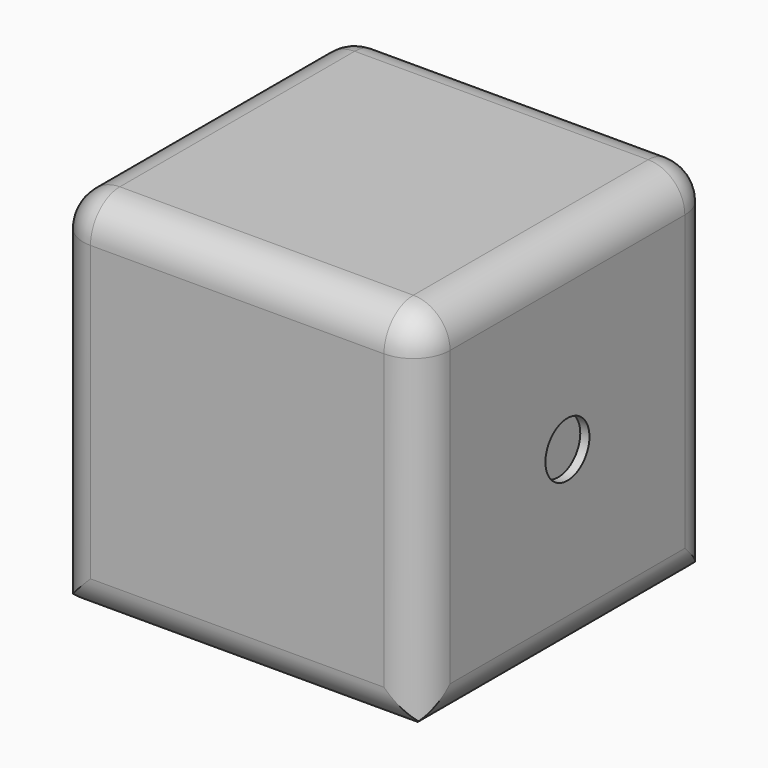
from build123d import *

# Parameters (mm, degrees)
F0_W         = 50.8
F0_H         = 50.8
F1_DEPTH     = 50.8
F2_R         = 5.08
F3_R         = 5.08
F4_T1_DEPTH  = 58.42
F4_T3_DEPTH  = 76.2
F4_T5_DEPTH  = 40.64
F4_S9_W      = 5.08
F4_S9_H      = 5.08
F4_T10_DEPTH = 5.08
F4_S15_W     = 5.08
F4_S15_H     = 5.08
F4_T16_DEPTH = 5.08
F4_T20_ANGLE = 90
F4_T22_ANGLE = 90
F5_T1_DEPTH  = 66.04
F6_T1_DEPTH  = 66.04
F7_R         = 3.81
F8_DEPTH     = 1.27


# Not quite as in the source:
# - a fillet or chamfer that OpenCascade refuses, or shapes differently, is made with other operations: its cross-section is extruded or revolved along the edge and cut away or added


with BuildPart() as f1:
    # F0 (on Front) → F1 (new body)
    with BuildSketch(Plane.XZ):
        with Locations((25.4, 25.4)):
            Rectangle(F0_W, F0_H)
    extrude(amount=F1_DEPTH)

    # F2
    f2_edges = [f1.edges().sort_by_distance(p)[0] for p in [
        (25.4, -50.8, 50.8),
    ]]
    fillet(f2_edges, radius=F2_R)

    # F3
    f3_edges = [f1.edges().sort_by_distance(p)[0] for p in [
        (25.4, 0, 50.8),
        (0, 0, 25.4),
        (25.4, 0, 0),
        (50.8, 0, 25.4),
    ]]
    fillet(f3_edges, radius=F3_R)

    # F4: fillet of radius 5.08 on 4 edges, made by hand

    # F4_s2 → F4_t1 (cut)
    with BuildSketch(Plane.XY.offset(-12.7)):
        with BuildLine():
            ThreePointArc((0, -45.72), (1.4878975516, -49.3121024484), (5.08, -50.8))
            Line((5.08, -50.8), (0, -50.8))
            Line((0, -50.8), (0, -45.72))
        make_face()
        with BuildLine():
            ThreePointArc((45.72, -50.8), (49.3121024484, -49.3121024484), (50.8, -45.72))
            Line((50.8, -45.72), (50.8, -50.8))
            Line((50.8, -50.8), (45.72, -50.8))
        make_face()
    extrude(amount=F4_T1_DEPTH, mode=Mode.SUBTRACT)

    # F4_s4 → F4_t3 (cut)
    with BuildSketch(Plane.YZ.offset(-12.7)):
        with BuildLine():
            ThreePointArc((-45.72, 0), (-49.3121024484, 1.4878975516), (-50.8, 5.08))
            Line((-50.8, 5.08), (-50.8, 0))
            Line((-50.8, 0), (-45.72, 0))
        make_face()
    extrude(amount=F4_T3_DEPTH, mode=Mode.SUBTRACT)

    # F4_s6 → F4_t5 (cut)
    with BuildSketch(Plane.XZ.offset(5.08)):
        with BuildLine():
            ThreePointArc((45.72, 50.8), (49.3121024484, 49.3121024484), (50.8, 45.72))
            Line((50.8, 45.72), (50.8, 50.8))
            Line((50.8, 50.8), (45.72, 50.8))
        make_face()
        with BuildLine():
            ThreePointArc((0, 45.72), (1.4878975516, 49.3121024484), (5.08, 50.8))
            Line((5.08, 50.8), (0, 50.8))
            Line((0, 50.8), (0, 45.72))
        make_face()
    extrude(amount=F4_T5_DEPTH, mode=Mode.SUBTRACT)


with BuildPart() as f4_tool8:
    # F4_s9 → F4_t10 (new body)
    with BuildSketch(Plane.XY.offset(45.72)):
        with Locations((48.26, -2.54)):
            Rectangle(F4_S9_W, F4_S9_H)
    extrude(amount=F4_T10_DEPTH)

    # F4_s11 → F4_t12 (revolve, cut)
    with BuildSketch(Plane(origin=(45.72, -5.08, 45.72), x_dir=(-0.7071067812, -0.7071067812, 0), z_dir=(-0.7071067812, 0.7071067812, 0))):
        with BuildLine():
            ThreePointArc((0, -5.08), (5.08, 0), (0, 5.08))
            Line((0, 5.08), (0, -5.08))
        make_face()
    revolve(axis=Axis((45.72, -5.08, 45.72), (0, 0, 1)), mode=Mode.SUBTRACT)


with BuildPart() as f1_1:
    add(f1.part)

    # F4_t7: cut F4_tool8
    add(f4_tool8.part, mode=Mode.SUBTRACT)


with BuildPart() as f4_tool14:
    # F4_s15 → F4_t16 (new body)
    with BuildSketch(Plane.YZ.offset(5.08)):
        with Locations((-2.54, 48.26)):
            Rectangle(F4_S15_W, F4_S15_H)
    extrude(amount=-F4_T16_DEPTH)

    # F4_s17 → F4_t18 (revolve, cut)
    with BuildSketch(Plane(origin=(5.08, -5.08, 45.72), x_dir=(0, -0.7071067812, -0.7071067812), z_dir=(0, 0.7071067812, -0.7071067812))):
        with BuildLine():
            ThreePointArc((0, -5.08), (5.08, 0), (0, 5.08))
            Line((0, 5.08), (0, -5.08))
        make_face()
    revolve(axis=Axis((5.08, -5.08, 45.72), (-1, 0, 0)), mode=Mode.SUBTRACT)


with BuildPart() as f1_2:
    add(f1_1.part)

    # F4_t13: cut F4_tool14
    add(f4_tool14.part, mode=Mode.SUBTRACT)

    # F4_s19 → F4_t20 (revolve, cut)
    with BuildSketch(Plane.XZ.offset(45.72)):
        with BuildLine():
            ThreePointArc((45.72, 50.8), (49.3121024484, 49.3121024484), (50.8, 45.72))
            Line((50.8, 45.72), (50.8, 50.8))
            Line((50.8, 50.8), (45.72, 50.8))
        make_face()
    revolve(axis=Axis((50.8, -45.72, 45.72), (1, 0, 0)), revolution_arc=F4_T20_ANGLE, mode=Mode.SUBTRACT)

    # F4_s21 → F4_t22 (revolve, cut)
    with BuildSketch(Plane.XZ.offset(45.72)):
        with BuildLine():
            ThreePointArc((0, 45.72), (1.4878975516, 49.3121024484), (5.08, 50.8))
            Line((5.08, 50.8), (0, 50.8))
            Line((0, 50.8), (0, 45.72))
        make_face()
    revolve(axis=Axis((0, -45.72, 45.72), (1, 0, 0)), revolution_arc=F4_T22_ANGLE, mode=Mode.SUBTRACT)

    # F5: fillet of radius 5.08 on 4 edges, made by hand

    # F5_s2 → F5_t1 (cut)
    with BuildSketch(Plane.XZ.offset(-7.62)):
        with BuildLine():
            ThreePointArc((0, 5.08), (1.4878975516, 1.4878975516), (5.08, 0))
            Line((5.08, 0), (0, 0))
            Line((0, 0), (0, 5.08))
        make_face()
    extrude(amount=F5_T1_DEPTH, mode=Mode.SUBTRACT)

    # F6: fillet of radius 5.08 on 4 edges, made by hand

    # F6_s2 → F6_t1 (cut)
    with BuildSketch(Plane.XZ.offset(-7.62)):
        with BuildLine():
            ThreePointArc((45.72, 0), (49.3121024484, 1.4878975516), (50.8, 5.08))
            Line((50.8, 5.08), (50.8, 0))
            Line((50.8, 0), (45.72, 0))
        make_face()
    extrude(amount=F6_T1_DEPTH, mode=Mode.SUBTRACT)

    # F7 (on face) → F8 (cut)
    with BuildSketch(Plane.YZ.offset(50.8)):
        with Locations((-25.4, 25.4)):
            Circle(F7_R)
    extrude(amount=-F8_DEPTH, mode=Mode.SUBTRACT)


solid = f1_2.part
